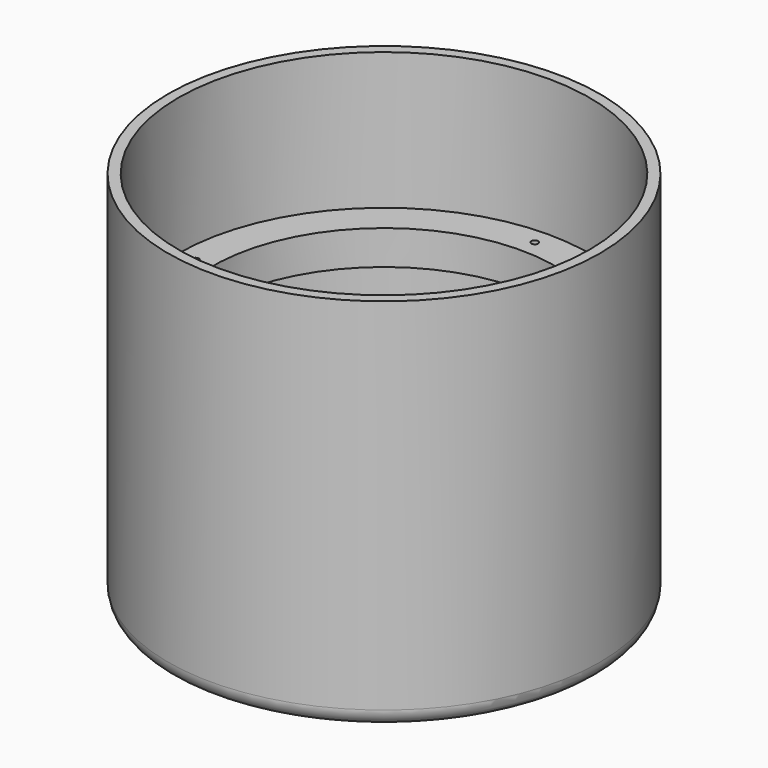
from build123d import *

# Parameters (mm, degrees)
F0_R     = 63
F0_R_2   = 60
F1_DEPTH = 40
F2_DEPTH = 70
F0_R_3   = 1
F0_R_4   = 50
F3_DEPTH = 10
F4_R     = 63
F4_R_2   = 60
F4_R_3   = 5
F5_DEPTH = 4
F6_R     = 5


with BuildPart() as f1:
    # F0 (on Top) → F1 (new body)
    with BuildSketch(Plane.XY):
        Circle(F0_R)
        Circle(F0_R_2, mode=Mode.SUBTRACT)
    extrude(amount=F1_DEPTH)

    # F0 (on Top) → F2 (join)
    with BuildSketch(Plane.XY):
        Circle(F0_R)
        Circle(F0_R_2, mode=Mode.SUBTRACT)
    extrude(amount=-F2_DEPTH)

    # F0 (on Top) → F3 (join)
    with BuildSketch(Plane.XY):
        Circle(F0_R_2)
        with Locations((0, -55)):
            Circle(F0_R_3, mode=Mode.SUBTRACT)
        with Locations((-55, 0)):
            Circle(F0_R_3, mode=Mode.SUBTRACT)
        Circle(F0_R_4, mode=Mode.SUBTRACT)
        with Locations((55, 0)):
            Circle(F0_R_3, mode=Mode.SUBTRACT)
        with Locations((0, 55)):
            Circle(F0_R_3, mode=Mode.SUBTRACT)
    extrude(amount=-F3_DEPTH)

    # F4 (on face) → F5 (join)
    with BuildSketch(Plane(origin=(0, 0, -70), x_dir=(1, 0, 0), z_dir=(0, 0, -1))):
        Circle(F4_R)
        Circle(F4_R_2, mode=Mode.SUBTRACT)
        Circle(F4_R_2)
        Circle(F4_R_3, mode=Mode.SUBTRACT)
    extrude(amount=-F5_DEPTH)

    # F6
    f6_edges = [f1.edges().sort_by_distance(p)[0] for p in [
        (-63, 0, -70),
        (-60, 0, -66),
    ]]
    fillet(f6_edges, radius=F6_R)


solid = f1.part
